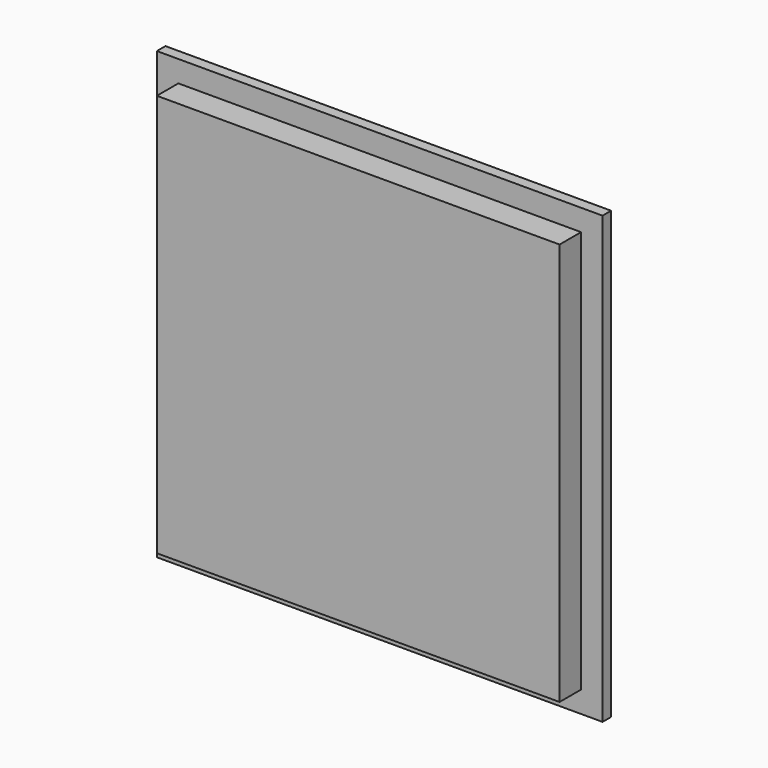
from build123d import *

# Parameters (mm, degrees)
F1_W     = 83
F1_H     = 83
F1_W_2   = 73
F1_H_2   = 73
F2_DEPTH = 2
F3_W     = 75
F3_H     = 75
F4_DEPTH = 5


# Not quite as in the source:
# - a feature names something its author has since deleted; it is built from what else it names


with BuildPart() as f2:
    # F1 (on Front) → F2 (new body)
    with BuildSketch(Plane.XZ):
        with Locations((-0.3727272727, 0)):
            Rectangle(F1_W, F1_H)
        with Locations((-0.3727272727, 0)):
            Rectangle(F1_W_2, F1_H_2, mode=Mode.SUBTRACT)
    extrude(amount=F2_DEPTH)

    # F3 (on face) → F4 (join)
    with BuildSketch(Plane.XZ.offset(2)):
        with Locations((-0.3727272727, 0)):
            Rectangle(F3_W, F3_H)
    extrude(amount=F4_DEPTH)


solid = f2.part
